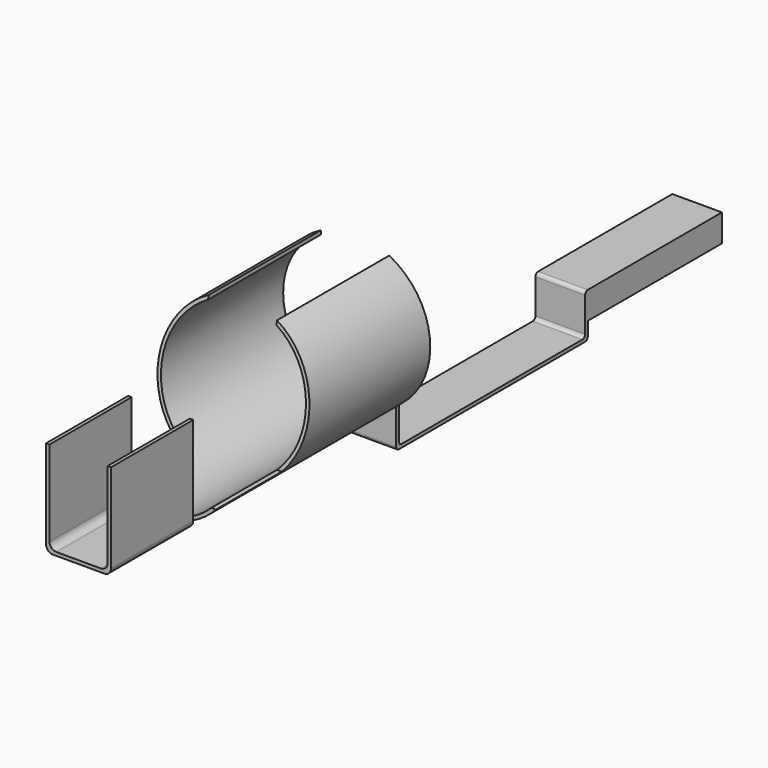
from build123d import *

# Parameters (mm, degrees)
F1_DEPTH     = 7.1
F2_W         = 1.45
F2_H         = 0.1
F3_DEPTH     = 0.6
F5_DEPTH     = 1.45
F6_R         = 0.1
F8_DEPTH     = 40
F10_DEPTH    = 3
F11_T1_DEPTH = 3
F11_T3_DEPTH = 4


# Not quite as in the source:
# - a fillet or chamfer that OpenCascade refuses, or shapes differently, is made with other operations: its cross-section is extruded or revolved along the edge and cut away or added


with BuildPart() as f1:
    # F0 (on Front) → F1 (new body)
    with BuildSketch(Plane.XZ):
        with BuildLine():
            Line((-1, 1.8466185313), (-1, 1.9595917942))
            ThreePointArc((-1, 1.9595917942), (0, -2.2), (1, 1.9595917942))
            Line((1, 1.9595917942), (1, 1.8466185313))
            ThreePointArc((1, 1.8466185313), (0, -2.1), (-1, 1.8466185313))
        make_face()
    extrude(amount=F1_DEPTH)

    # F2 (on face) → F3 (join)
    with BuildSketch(Plane(origin=(0, 0, 0), x_dir=(-1, 0, 0), z_dir=(0, 1, 0))):
        with Locations((0, -2.15)):
            Rectangle(F2_W, F2_H)
    extrude(amount=F3_DEPTH)

    # F4 (on face) → F5 (join, through all)
    with BuildSketch(Plane(origin=(-0.725, 0, 0), x_dir=(0, -1, 0), z_dir=(-1, 0, 0))):
        Polygon((-0.6, -3.4), (-0.6, -2.1), (-0.7, -2.1), (-0.7, -3.3), (-7.5, -3.3), (-7.5, -2.9), (-7.5, -2.1), (-12.5, -2.1), (-12.5, -2.9), (-7.6, -2.9), (-7.6, -3.4), align=None)
    extrude(amount=-F5_DEPTH)

    # F6
    f6_edges = [f1.edges().sort_by_distance(p)[0] for p in [
        (0, 0.7, -2.1),
        (0, 0.6, -2.2),
        (0, 0.6, -3.4),
        (0, 0.7, -3.3),
        (0, 7.5, -3.3),
        (0, 7.5, -2.1),
        (0, 7.6, -3.4),
    ]]
    fillet(f6_edges, radius=F6_R)

    # F7 (on Right) → F8 (cut, symmetric)
    with BuildSketch(Plane.YZ):
        Polygon((-4.7, -1.49), (-4.1, 1.9595917942), (-7.1, 1.9595917942), (-7.1, -1.49), align=None)
    extrude(amount=F8_DEPTH, both=True, mode=Mode.SUBTRACT)

    # F9 (on face) → F10 (join)
    with BuildSketch(Plane.XZ.offset(7.1)):
        Polygon((-0.95, 0.6), (-0.95, -2.2), (0.95, -2.2), (0.95, 0.6), (0.85, 0.6), (0.85, -2.1), (-0.85, -2.1), (-0.85, 0.6), align=None)
    extrude(amount=F10_DEPTH)

    # F11: fillet of radius 0.2 on 4 edges, made by hand

    # F11_s2 → F11_t1 (join)
    with BuildSketch(Plane.XZ.offset(7.1)):
        with BuildLine():
            ThreePointArc((-0.85, -1.9), (-0.7914213562, -2.0414213562), (-0.65, -2.1))
            Line((-0.65, -2.1), (-0.85, -2.1))
            Line((-0.85, -2.1), (-0.85, -1.9))
        make_face()
        with BuildLine():
            ThreePointArc((0.65, -2.1), (0.7914213562, -2.0414213562), (0.85, -1.9))
            Line((0.85, -1.9), (0.85, -2.1))
            Line((0.85, -2.1), (0.65, -2.1))
        make_face()
    extrude(amount=F11_T1_DEPTH)

    # F11_s4 → F11_t3 (cut)
    with BuildSketch(Plane.XZ.offset(6.6)):
        with BuildLine():
            ThreePointArc((-0.95, -2), (-0.8914213562, -2.1414213562), (-0.75, -2.2))
            Line((-0.75, -2.2), (-0.95, -2.2))
            Line((-0.95, -2.2), (-0.95, -2))
        make_face()
        with BuildLine():
            ThreePointArc((0.95, -2), (0.8914213562, -2.1414213562), (0.75, -2.2))
            Line((0.75, -2.2), (0.95, -2.2))
            Line((0.95, -2.2), (0.95, -2))
        make_face()
    extrude(amount=F11_T3_DEPTH, mode=Mode.SUBTRACT)


solid = f1.part
